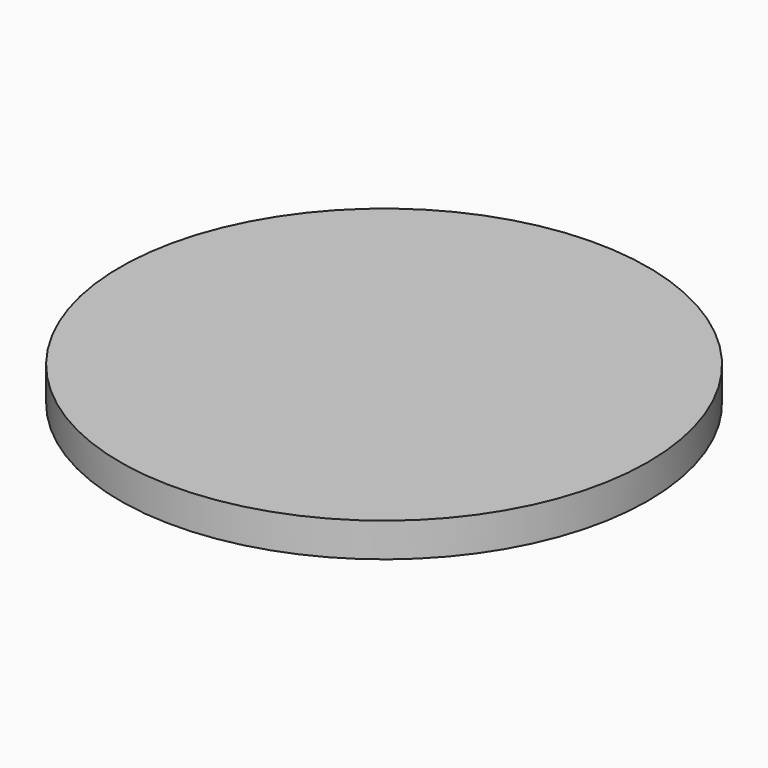
from build123d import *

# Parameters (mm, degrees)
F0_R     = 15.5
F1_DEPTH = 2


# Not quite as in the source:
# - the program builds the solid bodies; features that only make, move or delete a surface that nothing else refers to are left out


with BuildPart() as f1:
    # F0 (on Top) → F1 (new body)
    with BuildSketch(Plane.XY):
        Circle(F0_R)
    extrude(amount=F1_DEPTH)


solid = f1.part
